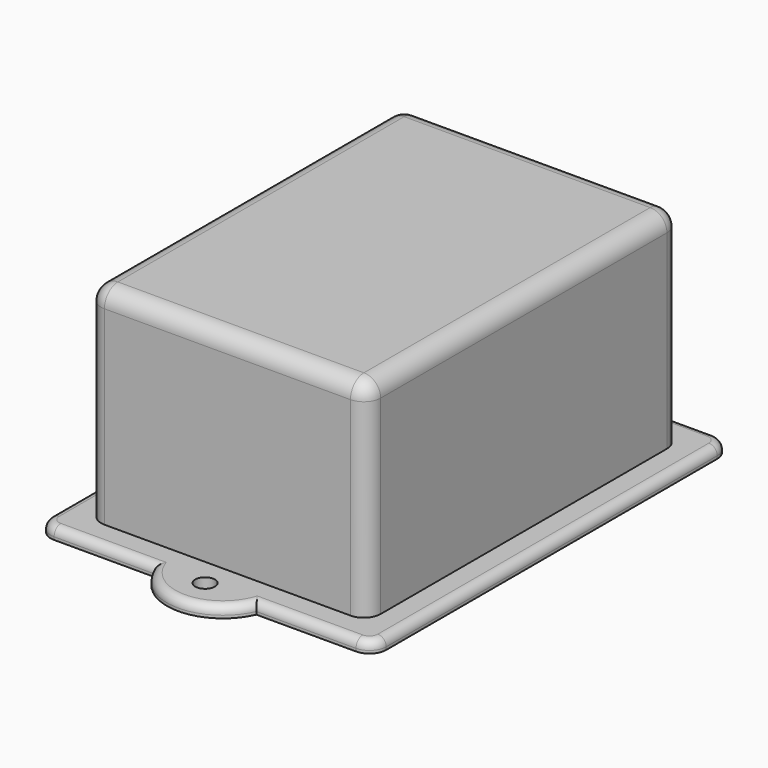
from build123d import *

# Parameters (mm, degrees)
F0_W     = 50
F0_H     = 70
F1_DEPTH = 37
F2_R     = 3
F3_T     = -2
F4_R     = 1.75
F5_DEPTH = 2
F6_R     = 1.5


# Not quite as in the source:
# - ends of sketch curves that miss each other by under 0.0002 mm in the source are joined
# - a feature names something its author has since deleted; it is built from what else it names


with BuildPart() as f1:
    # F0 (on Top) → F1 (new body)
    with BuildSketch(Plane.XY):
        Rectangle(F0_W, F0_H)
    extrude(amount=F1_DEPTH)

    # F2
    f2_edges = [f1.edges().sort_by_distance(p)[0] for p in [
        (25, 0, 37),
        (0, -35, 37),
        (25, -35, 18.5),
        (25, 35, 18.5),
        (0, 35, 37),
        (-25, 0, 37),
        (-25, -35, 18.5),
        (-25, 35, 18.5),
    ]]
    fillet(f2_edges, radius=F2_R)

    # F3
    f3_openings = [f1.faces().sort_by_distance(p)[0] for p in [
        (0, 0, 0),
    ]]
    offset(amount=F3_T, openings=f3_openings)


with BuildPart() as f5:
    # F4 (on Top) → F5 (new body)
    with BuildSketch(Plane.XY):
        with BuildLine():
            Line((9.1651513899, -40), (27, -40))
            ThreePointArc((27, -40), (29.1213201989, -39.1213204882), (30, -37.000000409))
            Line((30, -37.000000409), (30, 37.000000409))
            ThreePointArc((30, 37.000000409), (29.1213203436, 39.1213207526), (27, 40.000000409))
            Line((27, 40.000000409), (9.1651513899, 40))
            ThreePointArc((9.1651513899, 40), (0, 46), (-9.1651513899, 40))
            Line((-9.1651513899, 40), (-27, 40))
            ThreePointArc((-27, 40), (-29.1213202871, 39.121320809), (-30, 37.0000005686))
            Line((-30, 37.0000005686), (-30, -37.0000005686))
            ThreePointArc((-30, -37.0000005686), (-29.1213201425, -39.1213205446), (-27, -40))
            Line((-27, -40), (-9.1651513899, -40))
            ThreePointArc((-9.1651513899, -40), (0, -46), (9.1651513899, -40))
        make_face()
        with Locations((0, -40)):
            Circle(F4_R, mode=Mode.SUBTRACT)
        with Locations((0, 40)):
            Circle(F4_R, mode=Mode.SUBTRACT)
    extrude(amount=-F5_DEPTH)

    # F6
    f6_edges = [f5.edges().sort_by_distance(p)[0] for p in [
        (-30, 0, 0),
        (0, 46, 0),
        (18.082576, 40, 0),
        (29.12132, 39.121321, 0),
        (0, -46, 0),
    ]]
    fillet(f6_edges, radius=F6_R)


solid = Compound([f1.part, f5.part])
